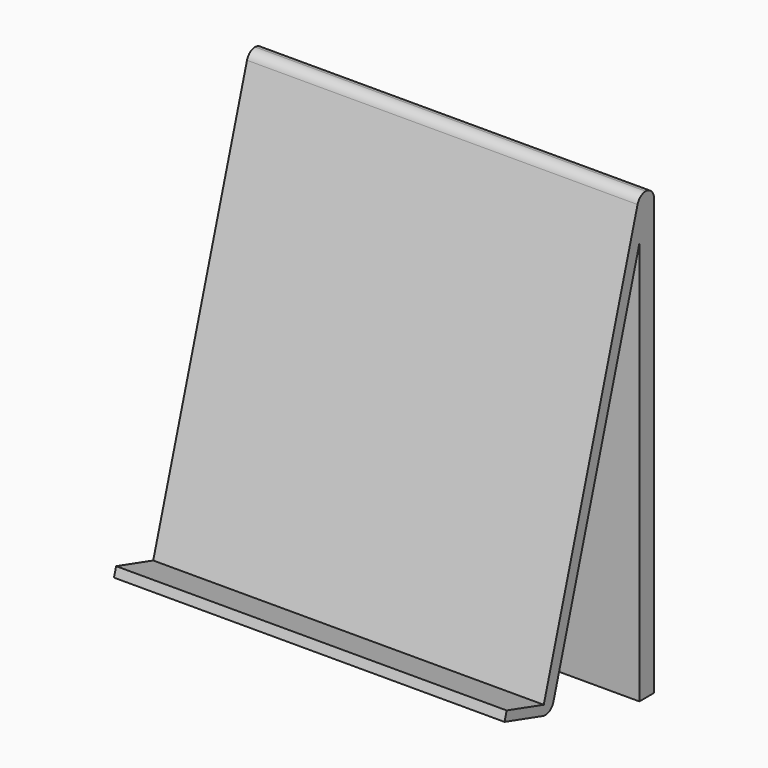
from build123d import *

# Parameters (mm, degrees)
F1_DEPTH      = 82.296
F1_DEPTH_BACK = 104.648
F2_R          = 5.08
F3_T1_DEPTH   = 205.8694200864
F4_R          = 5.08


# Not quite as in the source:
# - a fillet or chamfer that OpenCascade refuses, or shapes differently, is made with other operations: its cross-section is extruded or revolved along the edge and cut away or added


with BuildPart() as f1:
    # F0 (on Right) → F1 (new body, two sides)
    with BuildSketch(Plane.YZ) as f1_sk:
        Polygon((30.8638699353, 138.4397298098), (-26.3338502244, -53.1726228883), (-48.5219567113, -46.5493071791), (-49.8095880545, -50.8628719574), (-27.6214815676, -57.4861876667), (-22.003299054, -59.1632571598), (30.8638699353, 117.9417498623), (30.8638699353, -75.0317946076), (39.6366678178, -75.0317946076), (39.6366678178, 138.4397298098), align=None)
    extrude(amount=F1_DEPTH)
    extrude(f1_sk.sketch, amount=-F1_DEPTH_BACK)

    # F2
    f2_edges = [f1.edges().sort_by_distance(p)[0] for p in [
        (-11.176, 39.636668, 138.43973),
    ]]
    fillet(f2_edges, radius=F2_R)

    # F3: fillet of radius 5.08 on 1 edges, made by hand

    # F3_s2 → F3_t1 (cut)
    with BuildSketch(Plane.YZ.offset(-114.1107100432)):
        with BuildLine():
            ThreePointArc((34.6489539526, 138.4397298098), (31.6137560641, 137.4332999611), (29.7812013849, 134.8127903523))
            Line((29.7812013849, 134.8127903523), (30.8638699353, 138.4397298098))
            Line((30.8638699353, 138.4397298098), (34.6489539526, 138.4397298098))
        make_face()
    extrude(amount=F3_T1_DEPTH, mode=Mode.SUBTRACT)

    # F4
    f4_edges = [f1.edges().sort_by_distance(p)[0] for p in [
        (-11.176, -22.003299, -59.163257),
    ]]
    fillet(f4_edges, radius=F4_R)


solid = f1.part
